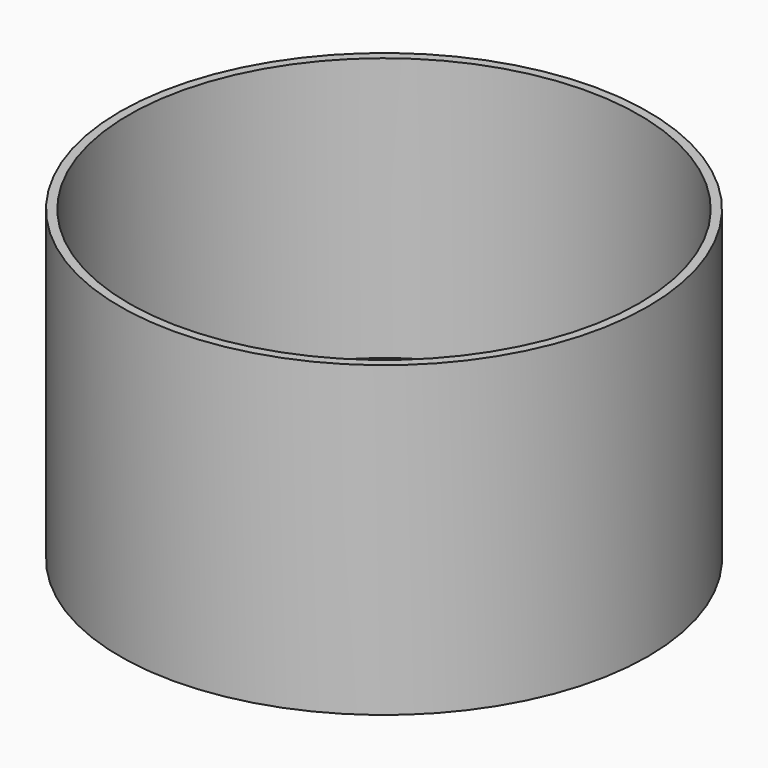
from build123d import *
from build123d import SkipClean  # not in build123d's __all__

# Parameters (mm, degrees)
F0_R     = 58
F1_DEPTH = 10
F0_R_2   = 60
F2_DEPTH = 70
F4_DEPTH = 10.001


with BuildPart() as f1:
    # F0 (on Top) → F1 (new body)
    with BuildSketch(Plane.XY):
        Circle(F0_R)
    extrude(amount=F1_DEPTH)

    # F0 (on Top) → F2 (join)
    with BuildSketch(Plane.XY):
        Circle(F0_R_2)
        Circle(F0_R, mode=Mode.SUBTRACT)
    extrude(amount=F2_DEPTH)

    # F3 (on face) → F4 (cut, through all)
    with BuildSketch(Plane.XY.offset(10)):
        with BuildLine():
            Line((-47.6370020393, 12.5), (-56.6370020393, 12.5))
            ThreePointArc((-56.6370020393, 12.5), (-58, 0), (-56.6370020393, -12.5))
            Line((-56.6370020393, -12.5), (-47.6370020393, -12.5))
            Line((-47.6370020393, -12.5), (-47.6370020393, 12.5))
        make_face()
    with SkipClean():  # cleaning this boolean's faces spoils the solid; the shape is the same uncleaned
        extrude(amount=-F4_DEPTH, mode=Mode.SUBTRACT)


solid = f1.part
